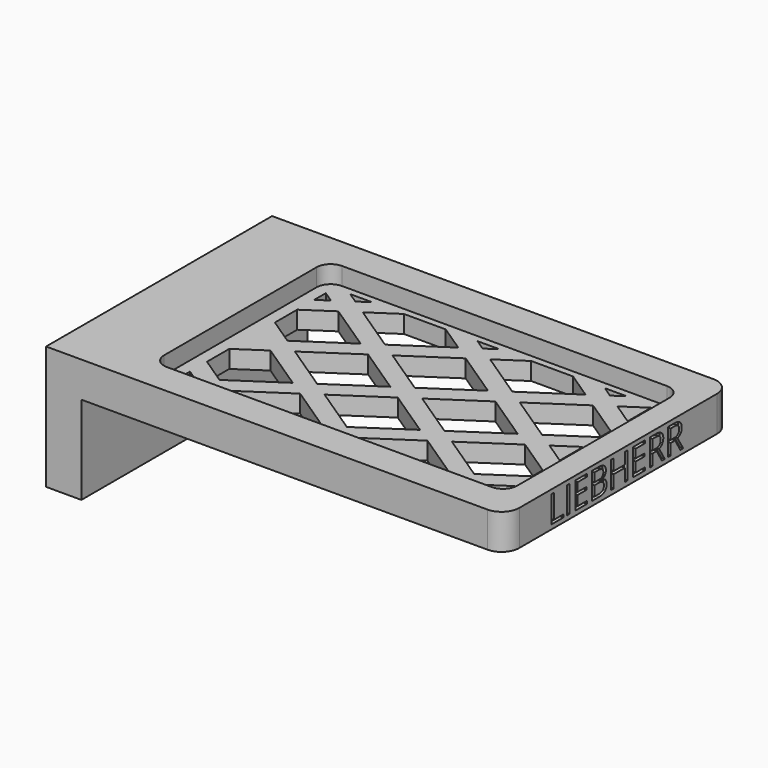
from build123d import *

# Parameters (mm, degrees)
F0_W         = 130
F0_H         = 80
F1_DEPTH     = 10
F3_DEPTH     = 5
F4_W         = 10
F4_H         = 80
F5_DEPTH     = 25
F6_TEXT_SIZE = 17.6953064097
F7_DEPTH     = 1
F8_TEXT_SIZE = 10.5610707899
F9_DEPTH     = 1
F11_DEPTH    = 25
F12_R        = 5


# Not quite as in the source:
# - Text() gives the source's letters only with a copy of the font that has no kerning and outlines rounded to 1/6400 em; it was checked with that copy


with BuildPart() as f1:
    # F0 (on Top) → F1 (new body)
    with BuildSketch(Plane.XY):
        with Locations((65, 40)):
            Rectangle(F0_W, F0_H)
    extrude(amount=F1_DEPTH)

    # F2 (on face) → F3 (cut)
    with BuildSketch(Plane.XY.offset(10)):
        with BuildLine():
            ThreePointArc((123, 67), (121.8284271247, 69.8284271247), (119, 71))
            Line((119, 71), (27, 71))
            ThreePointArc((27, 71), (24.1715728753, 69.8284271247), (23, 67))
            Line((23, 67), (23, 13))
            ThreePointArc((23, 13), (24.1715728753, 10.1715728753), (27, 9))
            Line((27, 9), (119, 9))
            ThreePointArc((119, 9), (121.8284271247, 10.1715728753), (123, 13))
            Line((123, 13), (123, 67))
        make_face()
    extrude(amount=-F3_DEPTH, mode=Mode.SUBTRACT)

    # F4 (on face) → F5 (join)
    with BuildSketch(Plane(origin=(0, 0, 0), x_dir=(1, 0, 0), z_dir=(0, 0, -1))):
        with Locations((5, -40)):
            Rectangle(F4_W, F4_H)
    extrude(amount=F5_DEPTH)

    # F6 (on face) → F7 (cut)
    with BuildSketch(Plane(origin=(0, 0, 0), x_dir=(0, -1, 0), z_dir=(-1, 0, 0))):
        with Locations((-80.4578493536, -18.8190411776)):
            Text('LIEBHERR', F6_TEXT_SIZE, font='Open Sans', text_align=(TextAlign.LEFT, TextAlign.BOTTOM))
    extrude(amount=-F7_DEPTH, mode=Mode.SUBTRACT)

    # F8 (on face) → F9 (cut)
    with BuildSketch(Plane.YZ.offset(130)):
        with Locations((15.3655496803, 1.25126075)):
            Text('LIEBHERR', F8_TEXT_SIZE, font='Open Sans', text_align=(TextAlign.LEFT, TextAlign.BOTTOM))
    extrude(amount=-F9_DEPTH, mode=Mode.SUBTRACT)

    # F10 (on face) → F11 (cut)
    with BuildSketch(Plane(origin=(0, 0, 0), x_dir=(1, 0, 0), z_dir=(0, 0, -1))):
        Polygon((33.9444872454, -61.0323824402), (47.4653045284, -52.0185042515), (33.9444872454, -43.0046260629), (26.3404008304, -48.0740170062), (26.3404008304, -55.9629914969), align=None)
        Polygon((57.8889744907, -69.1063994464), (65.4930609057, -64.0370085031), (51.9722436227, -55.0231303144), (38.4514263397, -64.0370085031), (46.0555127546, -69.1063994464), align=None)
        Polygon((70, -61.0323824402), (83.520817283, -52.0185042515), (70, -43.0046260629), (56.479182717, -52.0185042515), align=None)
        Polygon((33.9444872454, -36.9953739371), (47.4653045284, -27.9814957485), (33.9444872454, -18.9676175598), (26.3404008304, -24.0370085031), (26.3404008304, -31.9259829938), align=None)
        Polygon((38.4514263397, -15.9629914969), (51.9722436227, -24.9768696856), (65.4930609057, -15.9629914969), (57.8889744907, -10.8936005536), (46.0555127546, -10.8936005536), align=None)
        Polygon((51.9722436227, -49.0138781887), (65.4930609057, -40), (51.9722436227, -30.9861218113), (38.4514263397, -40), align=None)
        Polygon((56.479182717, -27.9814957485), (70, -36.9953739371), (83.520817283, -27.9814957485), (70, -18.9676175598), align=None)
        Polygon((74.5069390943, -15.9629914969), (88.0277563773, -24.9768696856), (101.5485736603, -15.9629914969), (93.9444872454, -10.8936005536), (82.1110255093, -10.8936005536), align=None)
        Polygon((110.562451849, -15.9629914969), (116.7797877734, -20.1078821132), (116.7797877734, -11.8181008806), align=None)
        Polygon((92.5346954716, -27.9814957485), (106.0555127546, -36.9953739371), (116.7797877734, -29.845857258), (116.7797877734, -26.1171342389), (106.0555127546, -18.9676175598), align=None)
        Polygon((74.5069390943, -40), (88.0277563773, -49.0138781887), (101.5485736603, -40), (88.0277563773, -30.9861218113), align=None)
        Polygon((110.562451849, -40), (116.7797877734, -44.1448906163), (116.7797877734, -35.8551093837), align=None)
        Polygon((92.5346954716, -52.0185042515), (106.0555127546, -61.0323824402), (116.7797877734, -53.8828657611), (116.7797877734, -50.154142742), (106.0555127546, -43.0046260629), align=None)
        Polygon((93.9444872454, -69.1063994464), (101.5485736603, -64.0370085031), (88.0277563773, -55.0231303144), (74.5069390943, -64.0370085031), (82.1110255093, -69.1063994464), align=None)
        Polygon((110.562451849, -64.0370085031), (116.7797877734, -68.1818991194), (116.7797877734, -59.8921178868), align=None)
        Polygon((102.958365434, -69.1063994464), (109.1526600753, -69.1063994464), (106.0555127546, -67.041634566), align=None)
        Polygon((30.8473399247, -69.1063994464), (37.041634566, -69.1063994464), (33.9444872454, -67.041634566), align=None)
        Polygon((26.3404008304, -66.1017733835), (29.437548151, -64.0370085031), (26.3404008304, -61.9722436227), align=None)
        Polygon((26.3404008304, -18.0277563773), (29.437548151, -15.9629914969), (26.3404008304, -13.8982266165), align=None)
        Polygon((30.8473399247, -10.8936005536), (33.9444872454, -12.958365434), (37.041634566, -10.8936005536), align=None)
        Polygon((102.958365434, -10.8936005536), (106.0555127546, -12.958365434), (109.1526600753, -10.8936005536), align=None)
        Polygon((66.9028526794, -69.1063994464), (73.0971473206, -69.1063994464), (70, -67.041634566), align=None)
        Polygon((66.9028526794, -10.8936005536), (70, -12.958365434), (73.0971473206, -10.8936005536), align=None)
    extrude(amount=-F11_DEPTH, mode=Mode.SUBTRACT)

    # F12
    f12_edges = [f1.edges().sort_by_distance(p)[0] for p in [
        (130, 0, 5),
        (130, 80, 5),
    ]]
    fillet(f12_edges, radius=F12_R)


solid = f1.part
